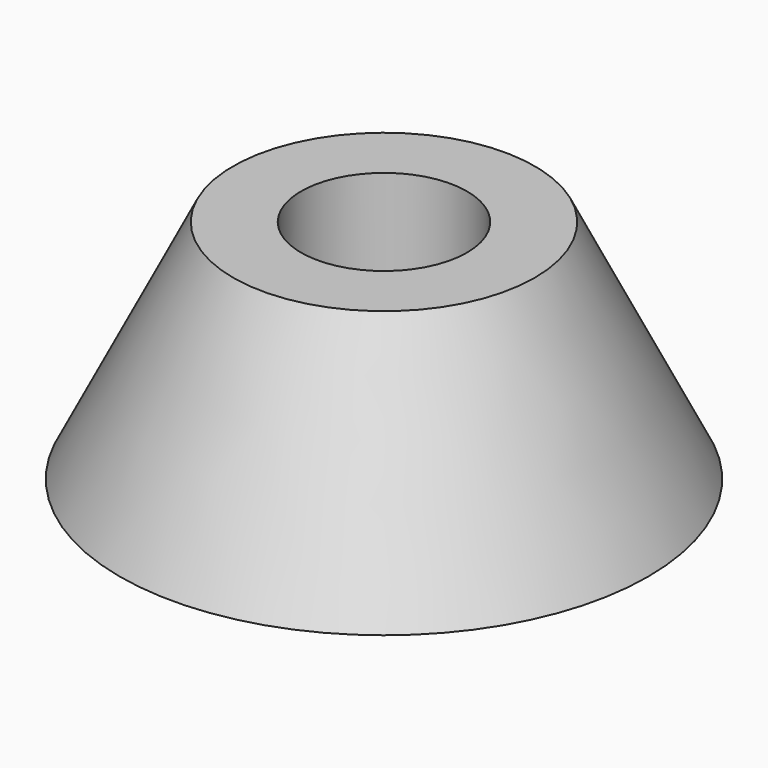
from build123d import *

# Parameters (mm, degrees)
F0_R     = 17.5
F0_R_2   = 10
F0_R_3   = 5.5
F1_DEPTH = 15
F2_SIZE2 = 14.99999
F2_SIZE  = 7.49999


# Not quite as in the source:
# - a fillet or chamfer is up to 0.001 mm smaller than in the source, because OpenCascade refuses the exact size


with BuildPart() as f1:
    # F0 (on Top) → F1 (new body)
    with BuildSketch(Plane.XY):
        Circle(F0_R)
        Circle(F0_R_2, mode=Mode.SUBTRACT)
        Circle(F0_R_2)
        Circle(F0_R_3, mode=Mode.SUBTRACT)
    extrude(amount=F1_DEPTH)

    # F2 (size 7.5 and 15 in the source; OpenCascade refuses exactly that, so slightly less here)
    f2_edges = [f1.edges().sort_by_distance(p)[0] for p in [
        (-17.5, 0, 15),
    ]]
    f2_side = f1.faces().sort_by_distance((-17.005025, 0, 15))[0]
    chamfer(f2_edges, length=F2_SIZE, length2=F2_SIZE2, reference=f2_side)


solid = f1.part
